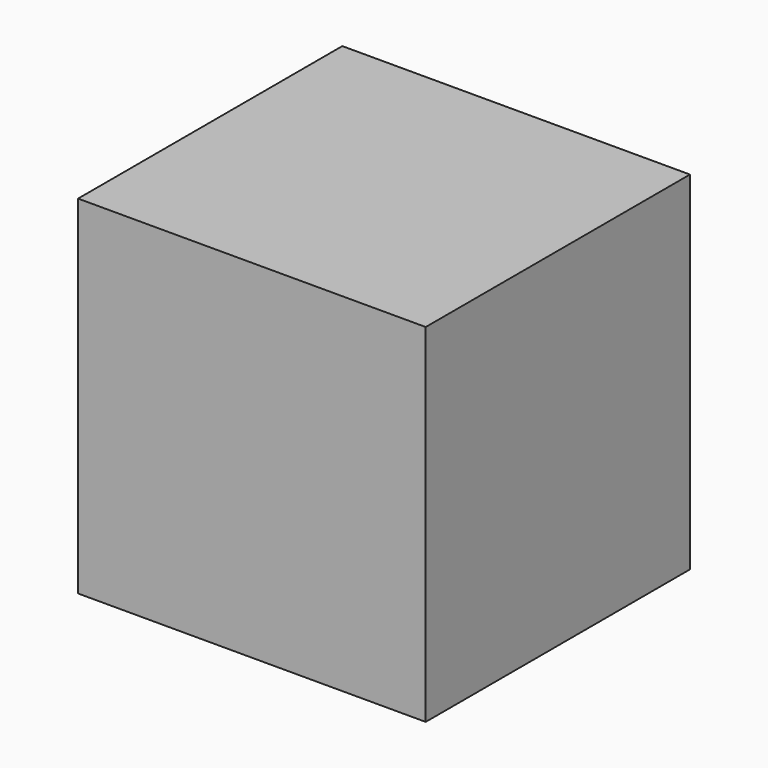
from build123d import *

# Parameters (mm, degrees)
F0_W     = 50
F0_H     = 50
F0_W_2   = 41
F0_H_2   = 40
F1_DEPTH = 47.5
F2_DEPTH = 45


# Not quite as in the source:
# - a feature names something its author has since deleted; it is built from what else it names


with BuildPart() as f1:
    # F0 (on Front) → F1 (new body)
    with BuildSketch(Plane.XZ):
        with Locations((-14.9696101435, 1.412372324)):
            Rectangle(F0_W, F0_H)
        with Locations((-14.9696101435, 1.912372324)):
            Rectangle(F0_W_2, F0_H_2, mode=Mode.SUBTRACT)
        with Locations((-14.9696101435, 1.912372324)):
            Rectangle(F0_W_2, F0_H_2)
    extrude(amount=F1_DEPTH)

    # F0 (on Front) → F2 (cut)
    with BuildSketch(Plane.XZ):
        with Locations((-14.9696101435, 1.912372324)):
            Rectangle(F0_W_2, F0_H_2)
    extrude(amount=F2_DEPTH, mode=Mode.SUBTRACT)


solid = f1.part
